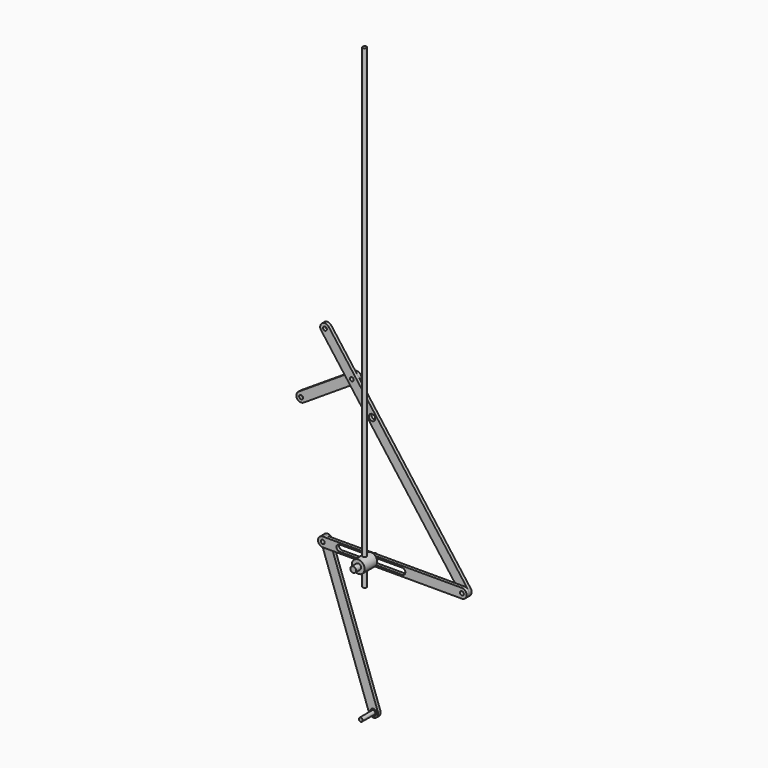
from build123d import *

# Parameters (mm, degrees)
F0_R          = 6
F1_DEPTH      = 1500
F2_R          = 20
F3_DEPTH      = 25
F3_DEPTH_BACK = 25
F4_R          = 9
F5_DEPTH      = 20
F6_R          = 9
F7_DEPTH      = 20
F8_R          = 6.1
F9_DEPTH      = 100
F11_DEPTH     = 10
F12_R         = 6.1
F13_DEPTH     = 25
F14_R         = 6.1
F15_DEPTH     = 25
F16_R         = 6.1
F17_DEPTH     = 10
F18_R         = 10
F18_R_2       = 6.1
F19_DEPTH     = 9.8
F20_R         = 10
F21_DEPTH     = 25
F22_R         = 6.1
F23_DEPTH     = 25
F25_DEPTH     = 10
F26_R         = 6
F27_DEPTH     = 50


with BuildPart() as f1:
    # F0 (on Top) → F1 (new body)
    with BuildSketch(Plane.XY):
        Circle(F0_R)
    extrude(amount=F1_DEPTH)


with BuildPart() as f3:
    # F2 (on Front) → F3 (new body, two sides)
    with BuildSketch(Plane.XZ) as f3_sk:
        with Locations((0, 66.0408288468)):
            Circle(F2_R)
    extrude(amount=F3_DEPTH)
    extrude(f3_sk.sketch, amount=-F3_DEPTH_BACK)

    # F4 (on face) → F5 (join)
    with BuildSketch(Plane.XZ.offset(25)):
        with Locations((0, 66.0408288468)):
            Circle(F4_R)
    extrude(amount=F5_DEPTH)

    # F6 (on face) → F7 (join)
    with BuildSketch(Plane(origin=(0, 25, 0), x_dir=(-1, 0, 0), z_dir=(0, 1, 0))):
        with Locations((0, 66.0408288468)):
            Circle(F6_R)
    extrude(amount=F7_DEPTH)

    # F8 (on Top) → F9 (cut)
    with BuildSketch(Plane.XY):
        Circle(F8_R)
    extrude(amount=F9_DEPTH, mode=Mode.SUBTRACT)


with BuildPart() as f11:
    # F10 (on face) → F11 (new body)
    with BuildSketch(Plane(origin=(0, 25, 0), x_dir=(-1, 0, 0), z_dir=(0, 1, 0))):
        with BuildLine():
            Line((152.0618690442, 80.1794555013), (-287.2134447098, 80.1794555079))
            ThreePointArc((-287.2134447098, 80.1794555079), (-302.210198455, 65.4915085567), (-287.8374157402, 50.1924391219))
            Line((-287.8374157402, 50.1924391219), (-286.5903583626, 50.192402315))
            Line((-286.5903583626, 50.192402315), (152.0618690442, 50.1794555144))
            Line((152.0618690442, 50.1794555144), (152.0618690442, 80.1794555013))
        make_face()
        with BuildLine():
            ThreePointArc((-98.8607928157, 55.3180821689), (-108.7221661547, 65.1794555079), (-98.8607928157, 75.0408288468))
            Line((-98.8607928157, 75.0408288468), (98.8607928157, 75.0408288468))
            ThreePointArc((98.8607928157, 75.0408288468), (108.7221661547, 65.1794555079), (98.8607928157, 55.3180821689))
            Line((98.8607928157, 55.3180821689), (-98.8607928157, 55.3180821689))
        make_face(mode=Mode.SUBTRACT)
        with BuildLine():
            Line((-286.5903583626, 50.192402315), (-287.8374157402, 50.1924391219))
            ThreePointArc((-287.8374157402, 50.1924391219), (-287.2138874341, 50.1794555144), (-286.5903583626, 50.192402315))
        make_face()
        with BuildLine():
            ThreePointArc((152.0618690442, 50.1794555144), (167.0623117685, 65.1794555079), (152.0618690442, 80.1794555013))
            Line((152.0618690442, 80.1794555013), (152.0618690442, 50.1794555144))
        make_face()
    extrude(amount=F11_DEPTH)

    # F12 (on face) → F13 (cut)
    with BuildSketch(Plane(origin=(0, 35, 0), x_dir=(-1, 0, 0), z_dir=(0, 1, 0))):
        with Locations((-287.2134447098, 65.1794555079)):
            Circle(F12_R)
    extrude(amount=-F13_DEPTH, mode=Mode.SUBTRACT)

    # F14 (on face) → F15 (cut)
    with BuildSketch(Plane(origin=(0, 35, 0), x_dir=(-1, 0, 0), z_dir=(0, 1, 0))):
        with Locations((152.0623117685, 65.1794555079)):
            Circle(F14_R)
    extrude(amount=-F15_DEPTH, mode=Mode.SUBTRACT)


with BuildPart() as f17:
    # F16 (on face) → F17 (new body)
    with BuildSketch(Plane(origin=(0, 35, 0), x_dir=(-1, 0, 0), z_dir=(0, 1, 0))):
        with BuildLine():
            Line((141.2023478455, 662.6265148895), (-298.9252010995, 74.5514756885))
            ThreePointArc((-298.9252010995, 74.5514756885), (-296.3940489054, 53.3170566525), (-275.2035315421, 56.1926882524))
            Line((-275.2035315421, 56.1926882524), (164.2665588229, 643.5003902394))
            Line((164.2665588229, 643.5003902394), (166.0567209766, 645.8927624252))
            ThreePointArc((166.0567209766, 645.8927624252), (161.588760798, 666.0813494708), (141.2023478455, 662.6265148895))
        make_face()
        with Locations((-287.2134447098, 65.1794555079)):
            Circle(F16_R, mode=Mode.SUBTRACT)
        with Locations((153.2114452098, 653.6386574978)):
            Circle(F16_R, mode=Mode.SUBTRACT)
        with BuildLine():
            Line((166.0567209766, 645.8927624252), (164.2665588229, 643.5003902394))
            ThreePointArc((164.2665588229, 643.5003902394), (165.2213583775, 644.6518902423), (166.0567209766, 645.8927624252))
        make_face()
    extrude(amount=F17_DEPTH)

    # F20 (on face) → F21 (cut)
    with BuildSketch(Plane(origin=(0, 45, 0), x_dir=(-1, 0, 0), z_dir=(0, 1, 0))):
        with Locations((4.4746835584, 454.9089351973)):
            Circle(F20_R)
    extrude(amount=-F21_DEPTH, mode=Mode.SUBTRACT)

    # F22 (on face) → F23 (cut)
    with BuildSketch(Plane(origin=(0, 45, 0), x_dir=(-1, 0, 0), z_dir=(0, 1, 0))):
        with Locations((68.5402597264, 540.5080434442)):
            Circle(F22_R)
    extrude(amount=-F23_DEPTH, mode=Mode.SUBTRACT)


with BuildPart() as f19:
    # F18 (on face) → F19 (new body)
    with BuildSketch(Plane(origin=(0, 35, 0), x_dir=(-1, 0, 0), z_dir=(0, 1, 0))):
        with BuildLine():
            Line((137.7026486797, 69.5153609467), (-14.1357335289, -358.208134007))
            ThreePointArc((-14.1357335289, -358.208134007), (-4.9357863724, -377.3908799351), (14.1931371418, -368.0795398482))
            Line((14.1931371418, -368.0795398482), (165.4493665169, 58.4128636653))
            Line((165.4493665169, 58.4128636653), (166.7213560809, 61.9994523872))
            ThreePointArc((166.7213560809, 61.9994523872), (156.513784022, 79.5037144687), (138.1828939866, 70.8681954417))
            Line((138.1828939866, 70.8681954417), (137.7026486797, 69.5153609467))
        make_face()
        with Locations((0, -363.2262051106)):
            Circle(F18_R, mode=Mode.SUBTRACT)
        with Locations((152.0623117685, 65.1794555079)):
            Circle(F18_R_2, mode=Mode.SUBTRACT)
        with BuildLine():
            ThreePointArc((138.1828939866, 70.8681954417), (137.9265782397, 70.1975266114), (137.7026486797, 69.5153609467))
            Line((137.7026486797, 69.5153609467), (138.1828939866, 70.8681954417))
        make_face()
        with BuildLine():
            Line((166.7213560809, 61.9994523872), (165.4493665169, 58.4128636653))
            ThreePointArc((165.4493665169, 58.4128636653), (166.1995612463, 60.1656568279), (166.7213560809, 61.9994523872))
        make_face()
    extrude(amount=F19_DEPTH)


with BuildPart() as f25:
    # F24 (on face) → F25 (new body)
    with BuildSketch(Plane(origin=(0, 45, 0), x_dir=(-1, 0, 0), z_dir=(0, 1, 0))):
        with BuildLine():
            ThreePointArc((81.1418503879, 532.37171056), (82.9281688852, 536.2668089495), (83.5402597264, 540.5080434442))
            ThreePointArc((83.5402597264, 540.5080434442), (81.9041987858, 547.320174742), (77.3529086839, 552.6462977813))
            ThreePointArc((77.3529086839, 552.6462977813), (56.1655326255, 548.9854327343), (60.4044718845, 527.9061008879))
            ThreePointArc((60.4044718845, 527.9061008879), (71.6979908964, 525.8441853619), (81.1418503879, 532.37171056))
        make_face()
        with BuildLine():
            ThreePointArc((74.6402597264, 540.5080434442), (74.3913427843, 538.7832747497), (73.6649065954, 537.1992680713))
            ThreePointArc((73.6649065954, 537.1992680713), (62.6891766685, 542.2328121387), (74.6402597264, 540.5080434442))
        make_face(mode=Mode.SUBTRACT)
        with BuildLine():
            ThreePointArc((77.3529086839, 552.6462977813), (81.9041987858, 547.320174742), (83.5402597264, 540.5080434442))
            ThreePointArc((83.5402597264, 540.5080434442), (82.9281688852, 536.2668089495), (81.1418503879, 532.37171056))
            Line((81.1418503879, 532.37171056), (223.9598778841, 440.1599378729))
            ThreePointArc((223.9598778841, 440.1599378729), (233.4032298314, 446.6873537668), (244.69638401, 444.6261107073))
            Line((244.69638401, 444.6261107073), (77.3529086839, 552.6462977813))
        make_face()
        with BuildLine():
            Line((223.9598778841, 440.1599378729), (81.1418503879, 532.37171056))
            ThreePointArc((81.1418503879, 532.37171056), (71.6979908964, 525.8441853619), (60.4044718845, 527.9061008879))
            Line((60.4044718845, 527.9061008879), (228.0024563935, 419.7051914959))
            ThreePointArc((228.0024563935, 419.7051914959), (221.8461044591, 429.1153306197), (223.9598778841, 440.1599378729))
        make_face()
        with BuildLine():
            ThreePointArc((251.5614685455, 432.0236049888), (249.7338588367, 439.1991282461), (244.69638401, 444.6261107073))
            ThreePointArc((244.69638401, 444.6261107073), (233.4032298314, 446.6873537668), (223.9598778841, 440.1599378729))
            ThreePointArc((223.9598778841, 440.1599378729), (221.8461044591, 429.1153306197), (228.0024563935, 419.7051914959))
            ThreePointArc((228.0024563935, 419.7051914959), (243.5118216919, 418.7310284462), (251.5614685455, 432.0236049888))
        make_face()
        with BuildLine():
            ThreePointArc((242.6614685455, 432.0236049888), (234.836699851, 426.1725219309), (231.4368216765, 435.3323803617))
            ThreePointArc((231.4368216765, 435.3323803617), (238.28623724, 437.8746880467), (242.6614685455, 432.0236049888))
        make_face(mode=Mode.SUBTRACT)
    extrude(amount=F25_DEPTH)


with BuildPart() as f27:
    # F26 (on face) → F27 (new body)
    with BuildSketch(Plane.XZ.offset(-35)):
        with Locations((0, -363.2262051106)):
            Circle(F26_R)
    extrude(amount=F27_DEPTH)


solid = Compound([f1.part, f3.part, f11.part, f17.part, f19.part, f25.part, f27.part])
